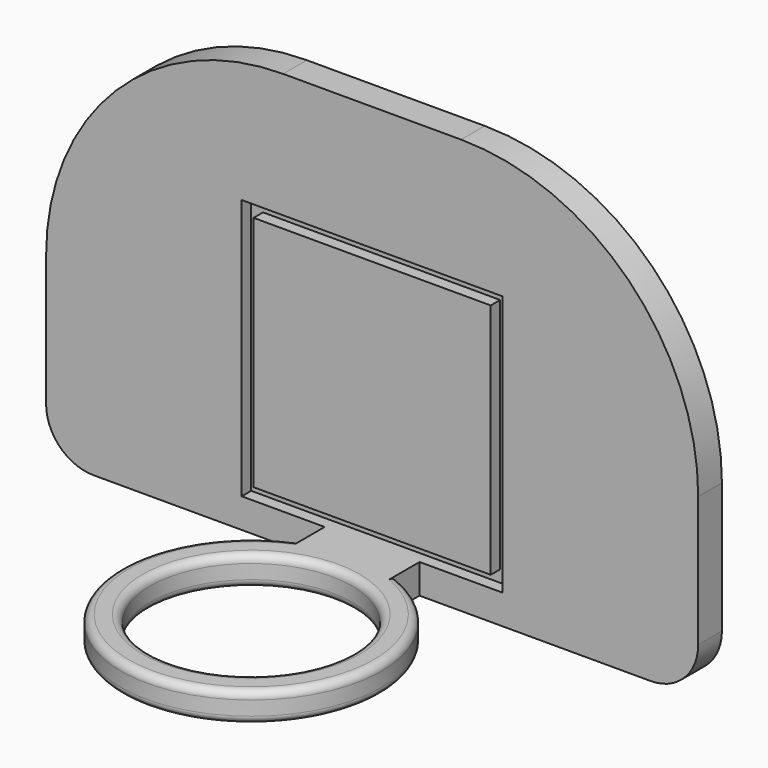
from build123d import *

# Parameters (mm, degrees)
F0_W      = 69.85
F0_H      = 44.45
F1_DEPTH  = 3.175
F2_R      = 25.4
F3_R      = 5.08
F4_W      = 10.16
F4_H      = 12.7
F5_DEPTH  = 25.4
F6_R      = 3.81
F7_DEPTH  = 19.05
F8_R      = 5.07999
F9_R      = 10.795
F10_DEPTH = 3.175
F11_R     = 0.8255
F12_W     = 27.94
F12_H     = 27.94
F12_W_2   = 25.4
F12_H_2   = 25.4
F13_DEPTH = 1.27


# Not quite as in the source:
# - a fillet or chamfer is up to 0.001 mm smaller than in the source, because OpenCascade refuses the exact size


with BuildPart() as f1:
    # F0 (on Front) → F1 (new body)
    with BuildSketch(Plane.XZ):
        with Locations((0, 22.225)):
            Rectangle(F0_W, F0_H)
    extrude(amount=F1_DEPTH)

    # F2
    f2_edges = [f1.edges().sort_by_distance(p)[0] for p in [
        (-34.925, -1.5875, 44.45),
        (34.925, -1.5875, 44.45),
    ]]
    fillet(f2_edges, radius=F2_R)

    # F3
    f3_edges = [f1.edges().sort_by_distance(p)[0] for p in [
        (-34.925, -1.5875, 0),
        (34.925, -1.5875, 0),
    ]]
    fillet(f3_edges, radius=F3_R)

    # F4 (on face) → F5 (join)
    with BuildSketch(Plane(origin=(0, 0, 0), x_dir=(1, 0, 0), z_dir=(0, 0, -1))):
        with Locations((0, -6.35)):
            Rectangle(F4_W, F4_H)
    extrude(amount=-F5_DEPTH)

    # F6 (on face) → F7 (cut)
    with BuildSketch(Plane(origin=(0, 0, 0), x_dir=(1, 0, 0), z_dir=(0, 0, -1))):
        with Locations((0, -6.35)):
            Circle(F6_R)
    extrude(amount=-F7_DEPTH, mode=Mode.SUBTRACT)

    # F8 (radius 5.08 in the source; OpenCascade refuses exactly that, so slightly less here)
    f8_edges = [f1.edges().sort_by_distance(p)[0] for p in [
        (-5.08, 12.7, 12.7),
        (5.08, 12.7, 12.7),
        (0, 0, 25.4),
        (-5.08, 6.35, 25.4),
        (0, 12.7, 25.4),
        (5.08, 6.35, 25.4),
        (5.08, 0, 12.7),
        (-5.08, 0, 12.7),
    ]]
    fillet(f8_edges, radius=F8_R)

    # F9 (on face) → F10 (join)
    with BuildSketch(Plane(origin=(0, 0, 0), x_dir=(1, 0, 0), z_dir=(0, 0, -1))):
        with BuildLine():
            Line((-5.08, 6.35), (-5.08, 3.175))
            Line((-5.08, 3.175), (5.08, 3.175))
            Line((5.08, 3.175), (5.08, 6.35))
            ThreePointArc((5.08, 6.35), (0, 33.3336274728), (-5.08, 6.35))
        make_face()
        with Locations((0, 19.3636274728)):
            Circle(F9_R, mode=Mode.SUBTRACT)
    extrude(amount=-F10_DEPTH)

    # F11
    f11_edges = [f1.edges().sort_by_distance(p)[0] for p in [
        (-10.795, -19.363627, 3.175),
        (0, -33.333627, 3.175),
        (0, -33.333627, 0),
        (-10.795, -19.363627, 0),
    ]]
    fillet(f11_edges, radius=F11_R)

    # F12 (on face) → F13 (cut)
    with BuildSketch(Plane.XZ.offset(3.175)):
        with Locations((0, 17.145)):
            Rectangle(F12_W, F12_H)
        with Locations((0, 17.145)):
            Rectangle(F12_W_2, F12_H_2, mode=Mode.SUBTRACT)
    extrude(amount=-F13_DEPTH, mode=Mode.SUBTRACT)


solid = f1.part
